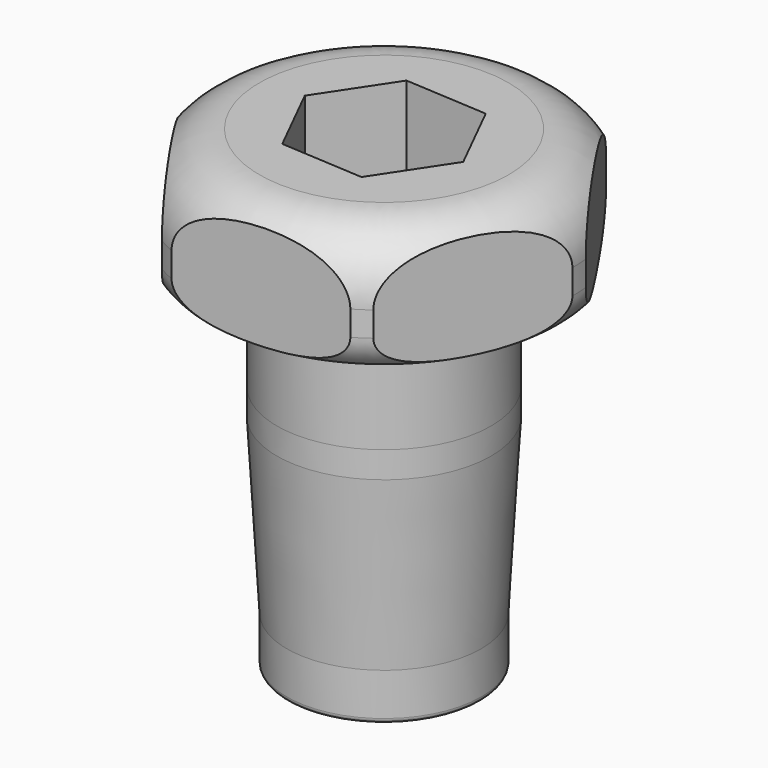
from build123d import *

# Parameters (mm, degrees)
F0_R         = 3.9
F2_DEPTH     = 14
F3_R         = 7.5
F4_DEPTH     = 5
F6_R         = 4.3
F7_DEPTH     = 4.1
F1_R         = 1.5693660879
F8_DEPTH     = 23.4
F9_DEPTH     = 15.5
F10_R        = 0.2
F11_S5_R     = 4.3
F11_T6_DEPTH = 9
F12_R        = 1.5
F13_R        = 2.5
F15_R        = 8.6051956913
F16_DEPTH    = 6


# Not quite as in the source:
# - a fillet or chamfer that OpenCascade refuses, or shapes differently, is made with other operations: its cross-section is extruded or revolved along the edge and cut away or added


with BuildPart() as f2:
    # F0 (on Top) → F2 (new body)
    with BuildSketch(Plane.XY):
        with Locations((-41.4718948305, -26.0946750641)):
            Circle(F0_R)
    extrude(amount=F2_DEPTH)

    # F3 (on face) → F4 (join)
    with BuildSketch(Plane.XY.offset(14)):
        with Locations((-41.4718948305, -26.0946750641)):
            Circle(F3_R)
    extrude(amount=F4_DEPTH)

    # F6 (on face) → F7 (join)
    with BuildSketch(Plane(origin=(0, 0, 14), x_dir=(1, 0, 0), z_dir=(0, 0, -1))):
        with Locations((-41.4718948305, 26.0946750641)):
            Circle(F6_R)
    extrude(amount=F7_DEPTH)

    # F1 (on Top) → F8 (cut)
    with BuildSketch(Plane.XY):
        with Locations((-41.495975107, -26.0728988796)):
            Circle(F1_R)
    extrude(amount=F8_DEPTH, mode=Mode.SUBTRACT)

    # F5 (on face) → F9 (cut)
    with BuildSketch(Plane.XY.offset(19)):
        Polygon((-39.9783341683, -29.0917753096), (-38.1295495491, -26.2997637113), (-39.6231102113, -23.3026634658), (-42.9654554927, -23.0975748186), (-44.8142401119, -25.8895864169), (-43.3206794497, -28.8866866624), align=None)
    extrude(amount=-F9_DEPTH, mode=Mode.SUBTRACT)

    # F10
    f10_edges = [f2.edges().sort_by_distance(p)[0] for p in [
        (-45.371895, -26.094675, 0),
    ]]
    fillet(f10_edges, radius=F10_R)

    # F11: chamfer of 8 x 0.4612770977 on 1 edges, made by hand


with BuildPart() as f11_tool2:
    # F11_s3 → F11_t4 (revolve)
    with BuildSketch(Plane.XZ.offset(26.0946750641)):
        Polygon((-37.5718948305, 1.9), (-37.1106177328, 9.9), (-37.5718948305, 9.9), align=None)
    revolve(axis=Axis((-41.4718948305, -26.0946750641, 9.9), (0, 0, -1)))

    # F11_s5 → F11_t6 (intersect, symmetric)
    with BuildSketch(Plane.XY.offset(5.9)):
        with Locations((-41.4718948305, -26.0946750641)):
            Circle(F11_S5_R)
    extrude(amount=F11_T6_DEPTH, both=True, mode=Mode.INTERSECT)


with BuildPart() as f2_1:
    add(f2.part)

    # F11_t1: union F11_tool2
    add(f11_tool2.part)

    # F12
    f12_edges = [f2_1.edges().sort_by_distance(p)[0] for p in [
        (-48.971895, -26.094675, 14),
    ]]
    fillet(f12_edges, radius=F12_R)

    # F13
    f13_edges = [f2_1.edges().sort_by_distance(p)[0] for p in [
        (-48.971895, -26.094675, 19),
    ]]
    fillet(f13_edges, radius=F13_R)

    # F15 (on face) → F16 (cut)
    with BuildSketch(Plane.XY.offset(19)):
        with Locations((-41.4718948305, -26.0946750641)):
            Circle(F15_R)
        Polygon((-49.1588137584, -26.5433145587), (-45.7038874939, -19.661927743), (-38.016968566, -19.2132882484), (-33.7849759026, -25.6460355695), (-37.2399021671, -32.5274223852), (-44.926821095, -32.9760618798), align=None, mode=Mode.SUBTRACT)
    extrude(amount=-F16_DEPTH, mode=Mode.SUBTRACT)


solid = f2_1.part
